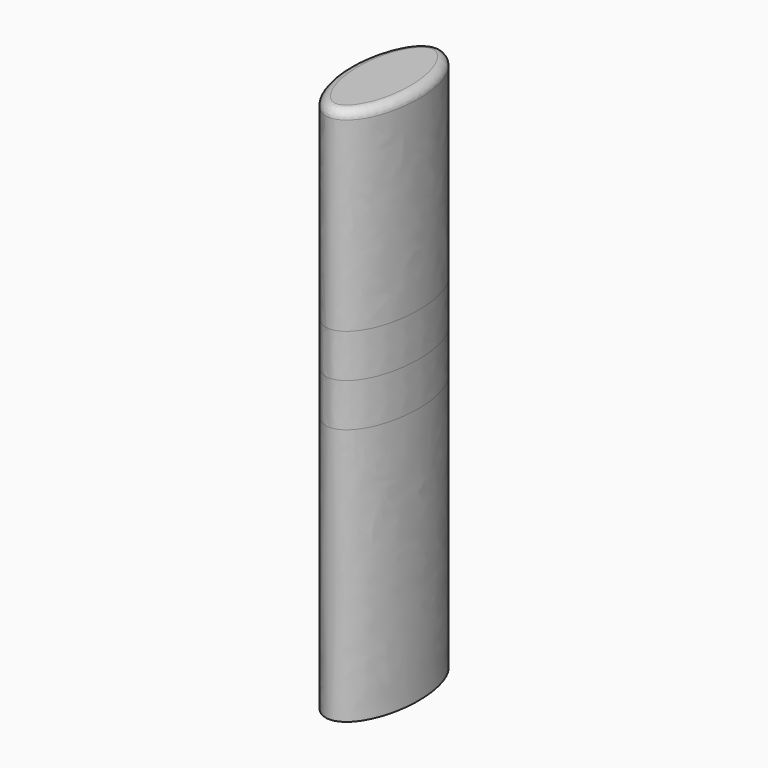
from build123d import *

# Parameters (mm, degrees)
F1_DEPTH = 25.4
F2_DEPTH = 114.046
F3_DEPTH = 25.4
F4_DEPTH = 150.622
F5_R     = 5.08


with BuildPart() as f1:
    # F0 (on Top) → F1 (new body)
    with BuildSketch(Plane.XY):
        with BuildLine():
            add(Edge.make_bspline(
                [(0, -13.0656813346), (35.1140165882, -13.0656813346), (17.5570082941, 46.9164226707), (0, 106.898526676), (-17.5570082941, 46.9164226707), (-35.1140165882, -13.0656813346), (0, -13.0656813346)],
                knots=[0, 0, 0, 2.0943951024, 2.0943951024, 4.1887902048, 4.1887902048, 6.2831853072, 6.2831853072, 6.2831853072], degree=2, weights=[1, 0.5, 1, 0.5, 1, 0.5, 1]))
        make_face()
    extrude(amount=F1_DEPTH)

    # F2 (add): faces of the model
    f2_faces = [f1.faces().sort_by_distance(p)[0] for p in [
        (0, 27.019379561, 25.4),
        (0, 27.019379561, 0),
    ]]
    extrude(f2_faces, amount=F2_DEPTH, dir=(0, 0, 1))

    # F3 (add): a face of the model
    f3_faces = [f1.faces().sort_by_distance(p)[0] for p in [
        (0, 27.019379561, 0),
    ]]
    extrude(f3_faces, amount=F3_DEPTH)

    # F4 (add): a face of the model
    f4_faces = [f1.faces().sort_by_distance(p)[0] for p in [
        (0, 27.019379561, -25.4),
    ]]
    extrude(f4_faces, amount=F4_DEPTH)

    # F5
    f5_edges = [f1.edges().sort_by_distance(p)[0] for p in [
        (4e-06, 66.910457, 139.446),
    ]]
    fillet(f5_edges, radius=F5_R)


solid = f1.part
